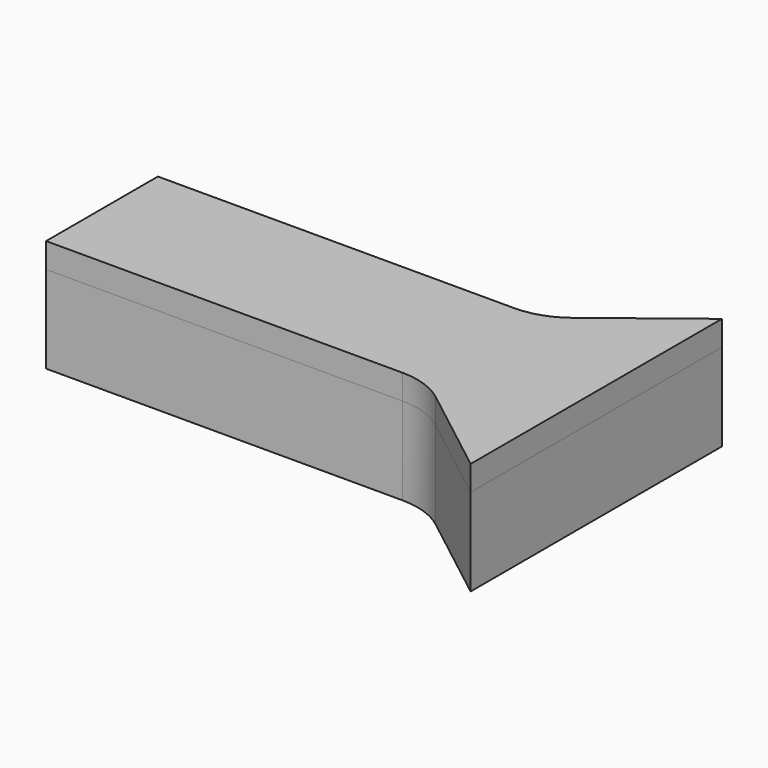
from build123d import *

# Parameters (mm, degrees)
F0_R     = 0.5
F1_DEPTH = 0.175
F2_R     = 0.3
F3_W     = 1.98
F3_H     = 3
F4_DEPTH = 0.5
F6_DEPTH = 0.1


# Not quite as in the source:
# - a feature of the source that left no trace in its solid (it failed there, or was rolled back) is left out


with BuildPart() as f1:
    # F0 (on Top) → F1 (new body, symmetric)
    with BuildSketch(Plane.XY):
        with BuildLine():
            Line((-7, 1.25), (-7, 0))
            Line((-7, 0), (-7, -1.25))
            Line((-7, -1.25), (-2.5, -1.25))
            Line((-2.5, -1.25), (-1.3311730507, -0.3429902873))
            ThreePointArc((-1.3311730507, -0.3429902873), (-1.2444571304, -0.2961841144), (-1.1472535137, -0.28))
            Line((-1.1472535137, -0.28), (0, -0.28))
            Line((0, -0.28), (1.1472535137, -0.28))
            ThreePointArc((1.1472535137, -0.28), (1.2444571304, -0.2961841144), (1.3311730507, -0.3429902873))
            Line((1.3311730507, -0.3429902873), (2.5, -1.25))
            Line((2.5, -1.25), (7, -1.25))
            Line((7, -1.25), (7, 0))
            Line((7, 0), (7, 1.25))
            Line((7, 1.25), (2.5, 1.25))
            Line((2.5, 1.25), (1.3311730507, 0.3429902873))
            ThreePointArc((1.3311730507, 0.3429902873), (1.2444571304, 0.2961841144), (1.1472535137, 0.28))
            Line((1.1472535137, 0.28), (0, 0.28))
            Line((0, 0.28), (-1.1472535137, 0.28))
            ThreePointArc((-1.1472535137, 0.28), (-1.2444571304, 0.2961841144), (-1.3311730507, 0.3429902873))
            Line((-1.3311730507, 0.3429902873), (-2.5, 1.25))
            Line((-2.5, 1.25), (-7, 1.25))
        make_face()
        with Locations((-5, 0)):
            Circle(F0_R, mode=Mode.SUBTRACT)
        with Locations((5, 0)):
            Circle(F0_R, mode=Mode.SUBTRACT)
    extrude(amount=F1_DEPTH, both=True)

    # F2
    f2_edges = [f1.edges().sort_by_distance(p)[0] for p in [
        (-2.5, -1.25, 0),
        (2.5, -1.25, 0),
        (-2.5, 1.25, 0),
        (2.5, 1.25, 0),
    ]]
    fillet(f2_edges, radius=F2_R)


with BuildPart() as f4:
    # F3 (on Top) → F4 (new body, symmetric)
    with BuildSketch(Plane.XY):
        with Locations((0.71, 0)):
            Rectangle(F3_W, F3_H)
    extrude(amount=F4_DEPTH, both=True)

    # F5: intersect F1
    add(f1.part, mode=Mode.INTERSECT)


with BuildPart() as f6:
    # F6 (new): a face of the model
    f6_faces = [f4.part.faces().sort_by_distance(p)[0] for p in [
        (0.8150350005, 0, 0.175),
    ]]
    extrude(f6_faces, amount=F6_DEPTH)


solid = Compound([f4.part, f6.part])
